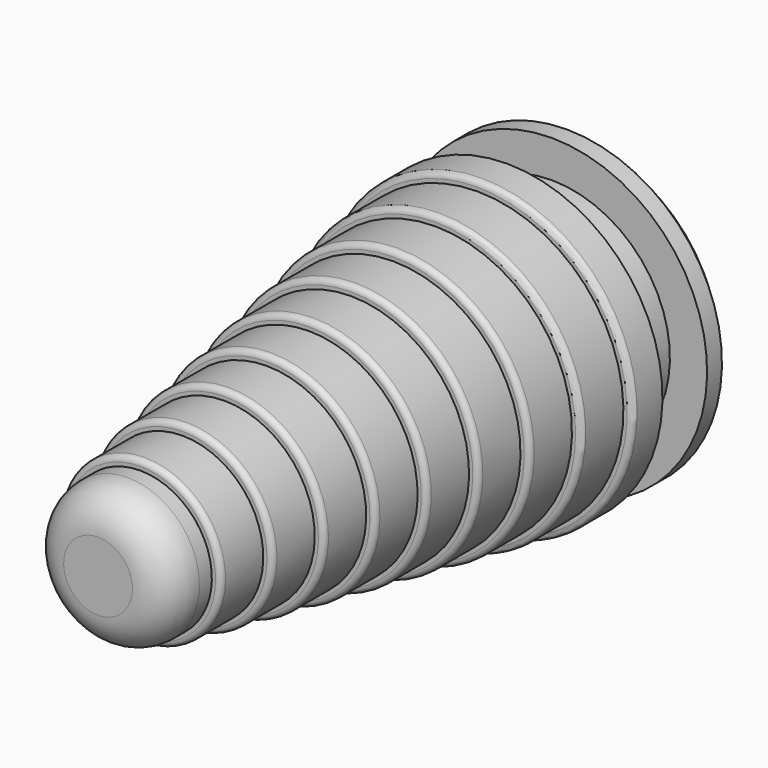
from build123d import *

# Parameters (mm, degrees)
F2_R     = 4.5
F3_DEPTH = 2
F4_R     = 2
F5_R     = 0.3
F6_SIZE  = 1
F7_T     = -1.2


# Not quite as in the source:
# - a shell that OpenCascade refuses in one call is made with other operations: the cavity is built on its own and cut out


with BuildPart() as f1:
    # F0 (on Right) → F1 (revolve)
    with BuildSketch(Plane.YZ):
        Polygon((-32.5, 0), (0, 0), (0, 8.35), (-2, 8.35), (-2, 6.35), (-5, 6.35), (-5, 8.35), (-7, 8.35), (-7, 7.85), (-9.8333333333, 7.85), (-9.8333333333, 7.35), (-12.6666666667, 7.35), (-12.6666666667, 6.85), (-15.5, 6.85), (-15.5, 6.35), (-18.3333333333, 6.35), (-18.3333333333, 5.85), (-21.1666666667, 5.85), (-21.1666666667, 5.35), (-24, 5.35), (-24, 4.85), (-26.8333333333, 4.85), (-26.8333333333, 4.35), (-29.6666666667, 4.35), (-29.6666666667, 3.85), (-32.5, 3.85), align=None)
    revolve(axis=Axis((0, -16.25, 0), (0, 1, 0)))

    # F2 (on face) → F3 (cut)
    with BuildSketch(Plane(origin=(0, 0, 0), x_dir=(-1, 0, 0), z_dir=(0, 1, 0))):
        Circle(F2_R)
    extrude(amount=-F3_DEPTH, mode=Mode.SUBTRACT)

    # F4
    f4_edges = [f1.edges().sort_by_distance(p)[0] for p in [
        (0, -32.5, -3.85),
    ]]
    fillet(f4_edges, radius=F4_R)

    # F5
    f5_edges = [f1.edges().sort_by_distance(p)[0] for p in [
        (0, -7, -8.35),
        (0, -9.833333, -7.85),
        (0, -12.666667, -7.35),
        (0, -15.5, -6.85),
        (0, -18.333333, -6.35),
        (0, -21.166667, -5.85),
        (0, -24, -5.35),
        (0, -26.833333, -4.85),
        (0, -29.666667, -4.35),
    ]]
    fillet(f5_edges, radius=F5_R)

    # F6
    f6_edges = [f1.edges().sort_by_distance(p)[0] for p in [
        (0, 0, -8.35),
    ]]
    chamfer(f6_edges, length=F6_SIZE)

    # F7: a shell. OpenCascade refuses it in one call, so the cavity is built on its own and cut out:
    # the body offset inwards by the wall thickness, plus a prism from it out through each open face.
    f7_core = offset(f1.part, amount=F7_T, kind=Kind.INTERSECTION, mode=Mode.PRIVATE)
    f7_exits = [f7_core.faces().sort_by_distance(p)[0] for p in [
        (0, -3.2, 0),
    ]]
    add(f7_core, mode=Mode.SUBTRACT)
    extrude(f7_exits, amount=-F7_T, mode=Mode.SUBTRACT)


solid = f1.part
